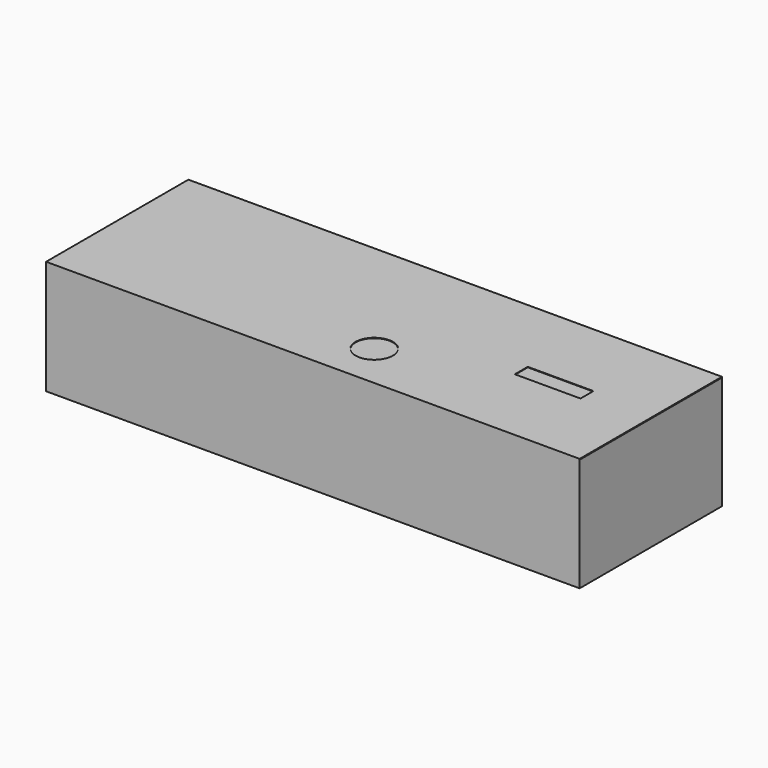
from build123d import *

# Parameters (mm, degrees)
F1_DEPTH = 209.55
F2_W     = 51.59375
F2_H     = 12.7
F3_DEPTH = 0.4064


# Not quite as in the source:
# - the dataset's text gives a spline's control points without its knots; the knots are read off the source's solid


with BuildPart() as f1:
    # F0 (on Right) → F1 (new body, symmetric)
    with BuildSketch(Plane.YZ):
        Polygon((-139.7, 0), (0, 0), (0, 88.9), (-139.2936, 88.9), (-139.2936, 89.154), (0, 89.154), (0, 89.5604), (-139.7, 89.5604), align=None)
    extrude(amount=F1_DEPTH, both=True)

    # F2 (on face) → F3 (cut, through all)
    with BuildSketch(Plane.XY.offset(89.5604)):
        with Locations((134.1027867572, -70.4335131599)):
            Rectangle(F2_W, F2_H)
        with BuildLine():
            add(Edge.make_bspline(
                [(30.1867131572, -93.7849015599), (27.4681765572, -91.0667205599), (23.6476101572, -89.4842243599), (19.8028375572, -89.4842243599)],
                knots=[7, 7, 7, 7, 8, 8, 8, 8], degree=3))
            add(Edge.make_bspline(
                [(19.8028375572, -89.4842243599), (15.9588015572, -89.4842243599), (12.1382351572, -91.0667205599), (9.4193175572, -93.7849015599)],
                knots=[0, 0, 0, 0, 1, 1, 1, 1], degree=3))
            add(Edge.make_bspline(
                [(9.4193175572, -93.7849015599), (6.7011365572, -96.5034127599), (5.1184625572, -100.3242077599), (5.1184625572, -104.1685993599), (5.1184625572, -108.0127877599), (6.7011365572, -111.8335827599), (9.4193175572, -114.5517637599)],
                knots=[1, 1, 1, 1, 2, 2, 2, 3, 3, 3, 3], degree=3))
            add(Edge.make_bspline(
                [(9.4193175572, -114.5517637599), (12.1382351572, -117.2702749599), (15.9588015572, -118.8529743599), (19.8028375572, -118.8529743599), (23.6476101572, -118.8529743599), (27.4681765572, -117.2702749599), (30.1867131572, -114.5517637599), (32.9049195572, -111.8335827599), (34.4872125572, -108.0127877599), (34.4872125572, -104.1685993599), (34.4872125572, -100.3242077599), (32.9049195572, -96.5034127599), (30.1867131572, -93.7849015599)],
                knots=[3, 3, 3, 3, 4, 4, 4, 5, 5, 5, 6, 6, 6, 7, 7, 7, 7], degree=3))
        make_face()
    extrude(amount=-F3_DEPTH, mode=Mode.SUBTRACT)


solid = f1.part
